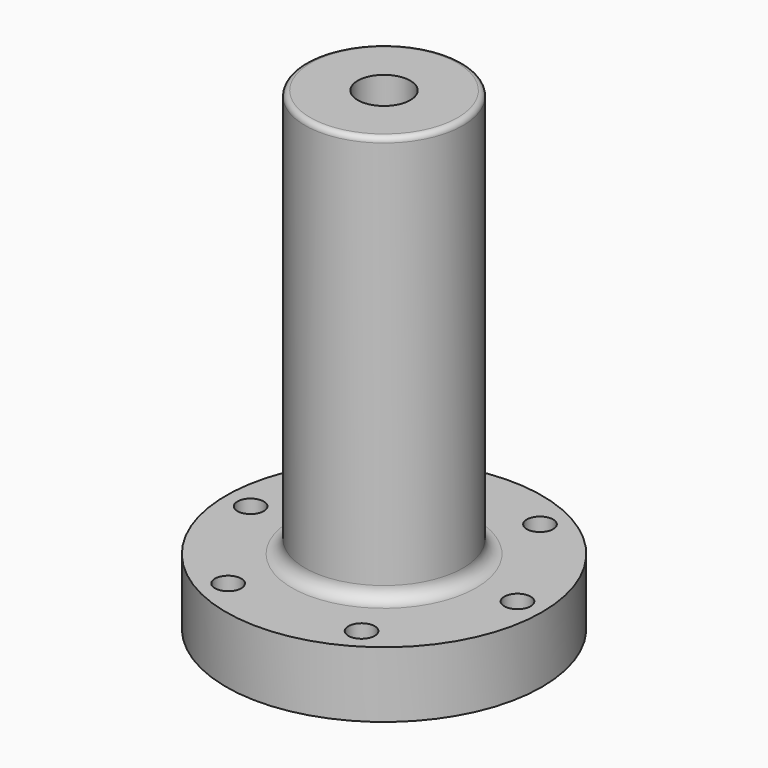
from build123d import *

# Parameters (mm, degrees)
F2_R          = 10
F3_DEPTH      = 145
F4_R          = 5
F5_DEPTH      = 25
F6_R          = 45
F6_R_2        = 40
F7_DEPTH      = 5
F8_R          = 5
F9_R          = 2
F10_R         = 2
F12_TEXT_SIZE = 34.7222222222
F13_DEPTH     = 1


# Not quite as in the source:
# - Text() gives the source's letters only with a copy of the font that has no kerning and outlines rounded to 1/6400 em; it was checked with that copy


with BuildPart() as f1:
    # F0 (on Front) → F1 (revolve)
    with BuildSketch(Plane.XZ):
        Polygon((188.8185292482, 97.6366343604), (158.8185292482, 97.6366343604), (158.8185292482, -82.3633656396), (218.8185292482, -82.3633656396), (218.8185292482, -57.3633656396), (188.8185292482, -57.3633656396), align=None)
    revolve(axis=Axis((158.8185292482, 0, 7.6366343604), (0, 0, -1)))

    # F2 (on face) → F3 (cut)
    with BuildSketch(Plane.XY.offset(97.6366343604)):
        with Locations((158.8185292482, 0)):
            Circle(F2_R)
    extrude(amount=-F3_DEPTH, mode=Mode.SUBTRACT)

    # F4 (on face) → F5 (cut)
    with BuildSketch(Plane.XY.offset(-57.3633656396)):
        with Locations((133.0665387718, 42.8671082852)):
            Circle(F4_R)
        with Locations((183.0665387718, 43.7354320932)):
            Circle(F4_R)
        with Locations((208.8185292482, 0.868323808)):
            Circle(F4_R)
        with Locations((184.5705197247, -42.8671082852)):
            Circle(F4_R)
        with Locations((108.8185292482, -0.868323808)):
            Circle(F4_R)
        with Locations((134.5705197247, -43.7354320932)):
            Circle(F4_R)
    extrude(amount=-F5_DEPTH, mode=Mode.SUBTRACT)

    # F6 (on face) → F7 (join)
    with BuildSketch(Plane(origin=(0, 0, -82.3633656396), x_dir=(1, 0, 0), z_dir=(0, 0, -1))):
        with Locations((158.8185292482, 0)):
            Circle(F6_R)
        with Locations((158.8185292482, 0)):
            Circle(F6_R_2, mode=Mode.SUBTRACT)
    extrude(amount=F7_DEPTH)

    # F8
    f8_edges = [f1.edges().sort_by_distance(p)[0] for p in [
        (128.818529, 0, -57.363366),
    ]]
    fillet(f8_edges, radius=F8_R)

    # F9
    f9_edges = [f1.edges().sort_by_distance(p)[0] for p in [
        (128.818529, 0, 97.636634),
    ]]
    fillet(f9_edges, radius=F9_R)

    # F10
    f10_edges = [f1.edges().sort_by_distance(p)[0] for p in [
        (113.818529, 0, -87.363366),
    ]]
    fillet(f10_edges, radius=F10_R)

    # F12 (on face) → F13 (join)
    with BuildSketch(Plane(origin=(0, 0, -82.3633656396), x_dir=(1, 0, 0), z_dir=(0, 0, -1))):
        with Locations((129.5711057054, -12.5)):
            Text('FTP', F12_TEXT_SIZE, font='Open Sans', text_align=(TextAlign.LEFT, TextAlign.BOTTOM))
    extrude(amount=F13_DEPTH)


solid = f1.part
